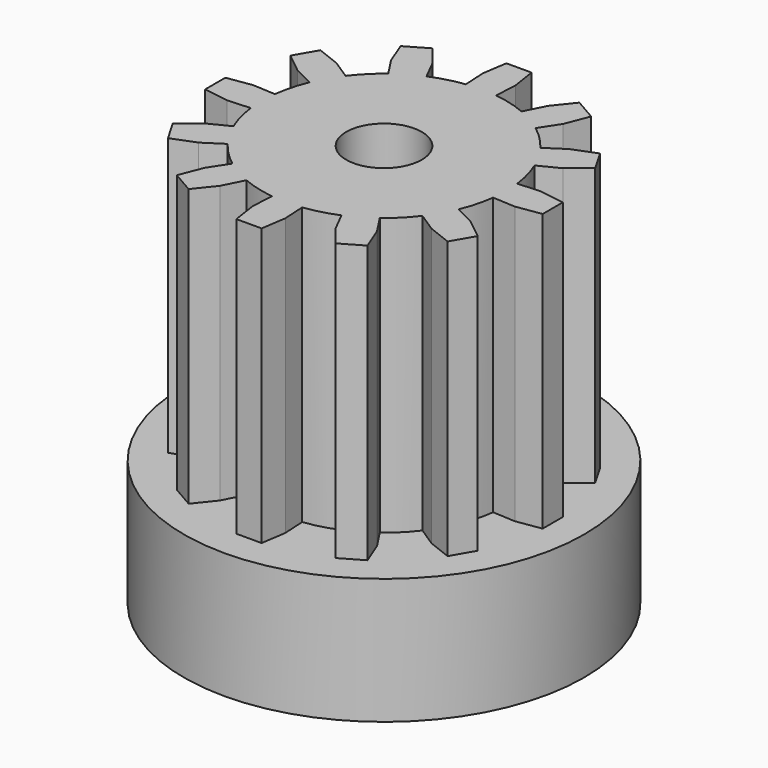
from build123d import *

# Parameters (mm, degrees)
F5_DEPTH        = 11
F5_COPIES_COUNT = 12


# Not quite as in the source:
# - a pattern or mirror of a feature is missing from the dataset's text; its kind, count and spacing are read off the source's solid


with BuildPart() as f1:
    # F0 (on Front) → F1 (revolve)
    with BuildSketch(Plane.XZ):
        Polygon((0, 16), (0, 0), (7.95, 0), (7.95, 5), (4.85, 5), (4.85, 16), align=None)
    revolve(axis=Axis((0, 0, 9.6948958626), (0, 0, 1)))

    # F2 (on Front) → F3 (revolve, cut)
    with BuildSketch(Plane.XZ):
        Polygon((0, 0), (2.7, 0), (2.7, 7.3), (1.5, 7.3), (1.5, 16), (0, 16), align=None)
    revolve(axis=Axis((0, 0, 9.4397878274), (0, 0, 1)), mode=Mode.SUBTRACT)

    # F4 (on face) → F5 (join, through all)
    with BuildSketch(Plane.XY.offset(16)):
        with BuildLine():
            Line((-0.65, 5.7127435003), (-0.6, 4.8127435003))
            ThreePointArc((-0.6, 4.8127435003), (0, 4.85), (0.6, 4.8127435003))
            Line((0.6, 4.8127435003), (0.65, 5.7127435003))
            Line((0.65, 5.7127435003), (0.5, 6.7))
            Line((0.5, 6.7), (-0.5, 6.7))
            Line((-0.5, 6.7), (-0.65, 5.7127435003))
        make_face()
    f5 = extrude(amount=-F5_DEPTH)

    # F5_copies: F5 ×12 about axis
    f5_copies_axis = Axis((0, 0, 0), (0, 0, 1))
    for i in range(1, F5_COPIES_COUNT):
        add(f5.rotate(f5_copies_axis, i * 360 / F5_COPIES_COUNT))


solid = f1.part
